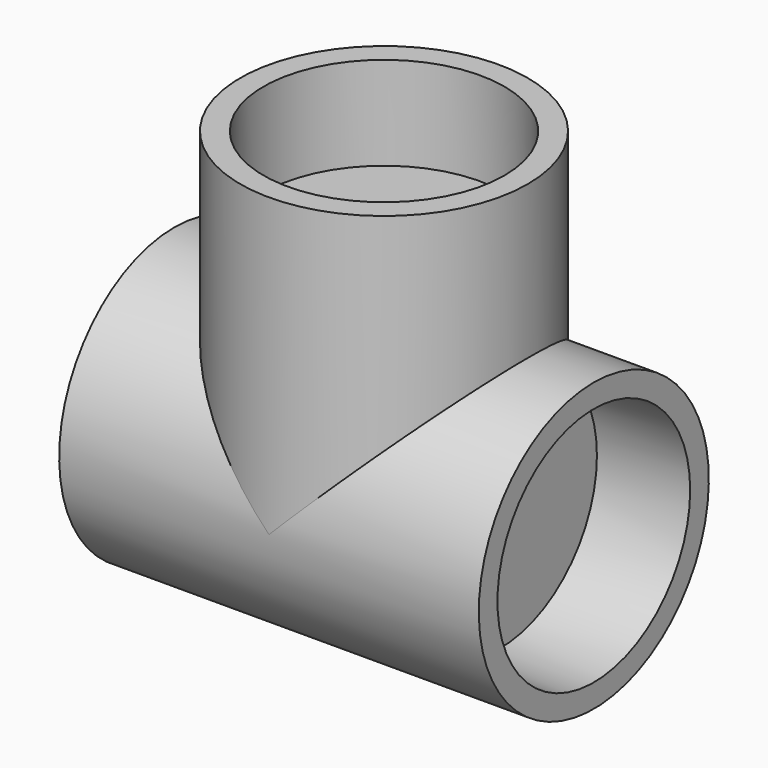
from build123d import *

# Parameters (mm, degrees)
F4_R     = 7.75
F5_DEPTH = 6
F6_R     = 7.75
F7_DEPTH = 6


# Not quite as in the source:
# - a pattern or mirror of a feature is missing from the dataset's text; its kind, count and spacing are read off the source's solid


with BuildPart() as f1:
    # F0 (on Front) → F1 (revolve)
    with BuildSketch(Plane.XZ):
        Polygon((13.5, 9.25), (0, 9.25), (-13.5, 9.25), (-13.5, 0), (0, 0), (13.5, 0), align=None)
    revolve(axis=Axis((6.75, 0, 0), (-1, 0, 0)))

    # F2 (on Front) → F3 (revolve)
    with BuildSketch(Plane.XZ):
        Polygon((9.25, 19.0967741935), (0, 19.0967741935), (0, 8.3548387097), (0, 0), (9.25, 0), (9.25, 8.3548387097), align=None)
    revolve(axis=Axis((0, 0, 13.7258064516), (0, 0, 1)))

    # F4 (on face) → F5 (cut)
    with BuildSketch(Plane.YZ.offset(13.5)):
        Circle(F4_R)
    f5 = extrude(amount=-F5_DEPTH, mode=Mode.SUBTRACT)

    # F5_copies: F5 across plane
    add(f5.mirror(Plane(origin=(0, 0, 0), x_dir=(0, 0, -1), z_dir=(-1, 0, 0))), mode=Mode.SUBTRACT)

    # F6 (on face) → F7 (cut)
    with BuildSketch(Plane.XY.offset(19.0967741935)):
        Circle(F6_R)
    extrude(amount=-F7_DEPTH, mode=Mode.SUBTRACT)


solid = f1.part
